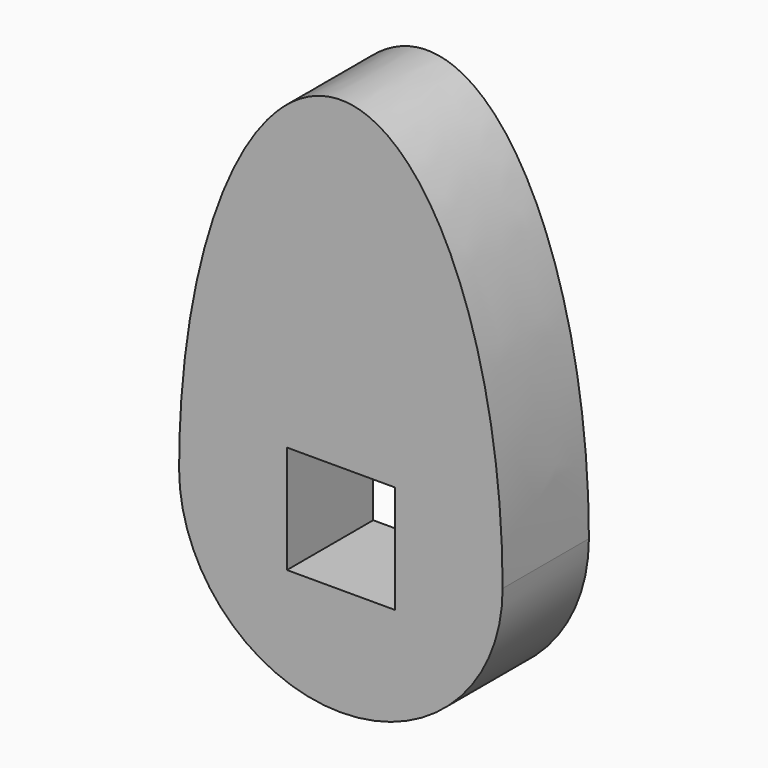
from build123d import *

# Parameters (mm, degrees)
F0_W     = 6.35
F0_H     = 6.35
F1_DEPTH = 6.35


with BuildPart() as f1:
    # F0 (on Front) → F1 (new body)
    with BuildSketch(Plane.XZ):
        with BuildLine():
            ThreePointArc((-9.525, -5.16e-08), (2.58e-08, -9.525), (9.525, 0))
            ThreePointArc((9.525, 0), (-2.58e-08, 9.525), (-9.525, -5.16e-08))
        make_face()
        Rectangle(F0_W, F0_H, mode=Mode.SUBTRACT)
        with BuildLine():
            ThreePointArc((-9.525, -5.16e-08), (-2.58e-08, 9.525), (9.525, 0))
            add(Edge.make_bspline(
                [(9.525, 0), (9.525, 22.2250000258), (-1.11e-08, 22.225), (-9.5250000221, 22.2249999742), (-9.525, -5.16e-08)],
                knots=[1.5707963268, 1.5707963268, 1.5707963268, 3.1415926548, 3.1415926548, 4.7123889827, 4.7123889827, 4.7123889827], degree=2, weights=[1, 0.7071067808, 1, 0.7071067808, 1]))
        make_face()
    extrude(amount=F1_DEPTH)


solid = f1.part
